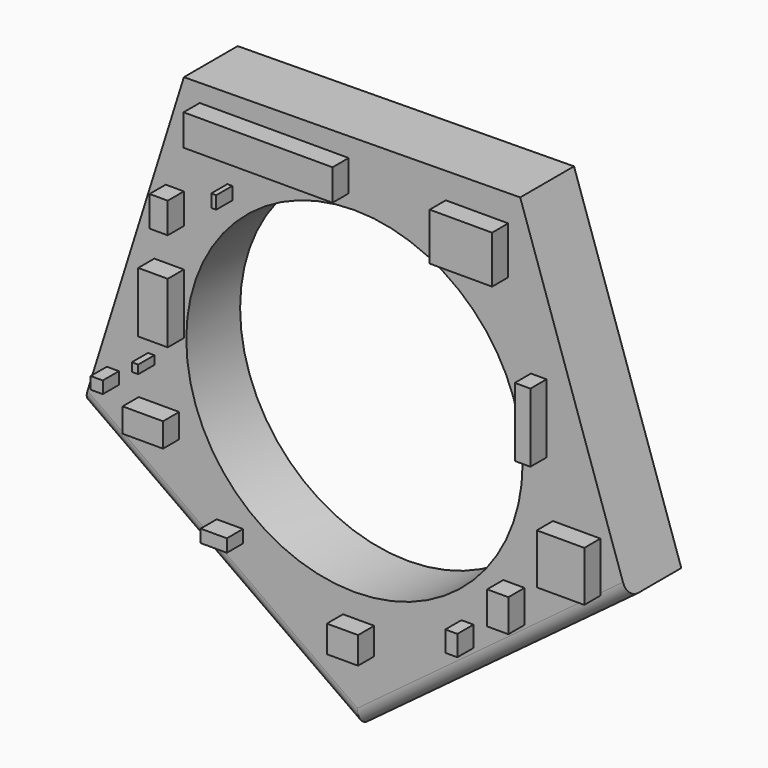
from build123d import *

# Parameters (mm, degrees)
F0_R         = 25
F1_DEPTH     = 10
F2_W         = 0.9488426149
F2_H         = 1.2651239522
F2_W_2       = 6.0093384236
F2_H_2       = 3.584517166
F2_W_3       = 3.9007980376
F2_H_3       = 1.8976870924
F2_W_4       = 4.6387878247
F2_H_4       = 4.0062256157
F2_W_5       = 1.7922576517
F2_H_5       = 3.0573830009
F2_W_6       = 7.0636067539
F2_H_6       = 7.4619053196
F2_W_7       = 3.1628105789
F2_H_7       = 4.8496406525
F2_W_8       = 2.3193918169
F2_H_8       = 10.2264162851
F2_W_9       = 9.2775728554
F2_H_9       = 7.0636067539
F2_W_10      = 22.1396633424
F2_H_10      = 4.6387854964
F2_W_11      = 2.7022243196
F2_H_11      = 4.5333597809
F2_W_12      = 0.7379893214
F2_H_12      = 1.8976833671
F2_W_13      = 4.3890562559
F2_H_13      = 8.9737139642
F2_W_14      = 1.7922595143
F2_H_14      = 1.7922581173
F3_DEPTH     = 3
F4_T1_DEPTH  = 60
F4_T6_DEPTH  = 60
F4_T12_DEPTH = 60
F4_T18_DEPTH = 60


# Not quite as in the source:
# - a fillet or chamfer that OpenCascade refuses, or shapes differently, is made with other operations: its cross-section is extruded or revolved along the edge and cut away or added


with BuildPart() as f1:
    # F0 (on Front) → F1 (new body)
    with BuildSketch(Plane.XZ):
        Polygon((-25.3573476618, 34.1470630352), (-40.3116381718, -13.5642479438), (0.4433851295, -42.5302292964), (40.5856652519, -12.7208793106), (24.6399354522, 34.6682935156), align=None)
        Circle(F0_R, mode=Mode.SUBTRACT)
    extrude(amount=F1_DEPTH)

    # F2 (on face) → F3 (join)
    with BuildSketch(Plane.XZ.offset(10)):
        with Locations((-30.2208252251, -4.310084274)):
            Rectangle(F2_W, F2_H)
        with Locations((-29.0611283854, -11.6899730638)):
            Rectangle(F2_W_2, F2_H_2)
        with Locations((-18.5184301808, -23.0760863051)):
            Rectangle(F2_W_3, F2_H_3)
        with Locations((0.6165653467, -30.455974862)):
            Rectangle(F2_W_4, F2_H_4)
        with Locations((16.7996054515, -25.0264853239)):
            Rectangle(F2_W_5, F2_H_5)
        with Locations((33.0353630707, -9.833295284)):
            Rectangle(F2_W_6, F2_H_6)
        with Locations((23.7050717697, -18.6481522396)):
            Rectangle(F2_W_7, F2_H_7)
        with Locations((27.3950155824, 7.0233154693)):
            Rectangle(F2_W_8, F2_H_8)
        with Locations((18.2228693739, 27.1598668769)):
            Rectangle(F2_W_9, F2_H_9)
        with Locations((-11.9292445015, 29.2156925425)):
            Rectangle(F2_W_10, F2_H_10)
        with Locations((-26.7084598216, 16.9334514067)):
            Rectangle(F2_W_11, F2_H_11)
        with Locations((-18.5184301808, 21.3086707518)):
            Rectangle(F2_W_12, F2_H_12)
        with Locations((-27.5518757897, 4.4868569821)):
            Rectangle(F2_W_13, F2_H_13)
        with Locations((-35.9138809144, -8.3690227475)):
            Rectangle(F2_W_14, F2_H_14)
    extrude(amount=F3_DEPTH)

    # F4: fillet of radius 2 on 2 edges, made by hand

    # F4_s2 → F4_t1 (cut)
    with BuildSketch(Plane(origin=(-24.4530139807, 0, 17.3795888115), x_dir=(0, 1, 0), z_dir=(0.815100466, 0, -0.5793196271))):
        with BuildLine():
            ThreePointArc((-8, -34.4095480118), (-9.4142135624, -33.8237615742), (-10, -32.4095480118))
            Line((-10, -32.4095480118), (-10, -34.4095480118))
            Line((-10, -34.4095480118), (-8, -34.4095480118))
        make_face()
    extrude(amount=F4_T1_DEPTH, mode=Mode.SUBTRACT)


with BuildPart() as f4_tool4:
    # F4_s5 → F4_t6 (new body)
    with BuildSketch(Plane(origin=(-24.0853680735, 0, -17.8856099914), x_dir=(0, 1, 0), z_dir=(0.8028456024, 0, 0.5961869997))):
        with BuildLine():
            ThreePointArc((-10, -32.4095480118), (-9.4142135624, -33.8237615742), (-8, -34.4095480118))
            Line((-8, -34.4095480118), (-10, -34.4095480118))
            Line((-10, -34.4095480118), (-10, -32.4095480118))
        make_face()
    extrude(amount=F4_T6_DEPTH)

    split(bisect_by=Plane.XY.offset(-13.5642479438), keep=Keep.BOTTOM)

    split(bisect_by=Plane.YZ.offset(36.5671664476), keep=Keep.BOTTOM)


with BuildPart() as f1_1:
    add(f1.part)

    # F4_t3: cut F4_tool4
    add(f4_tool4.part, mode=Mode.SUBTRACT)


with BuildPart() as f4_tool10:
    # F4_s11 → F4_t12 (new body)
    with BuildSketch(Plane(origin=(-24.0853680735, 0, -17.8856099914), x_dir=(0, 1, 0), z_dir=(0.8028456024, 0, 0.5961869997))):
        with BuildLine():
            ThreePointArc((-10, -32.4095480118), (-9.4142135624, -33.8237615742), (-8, -34.4095480118))
            Line((-8, -34.4095480118), (-10, -34.4095480118))
            Line((-10, -34.4095480118), (-10, -32.4095480118))
        make_face()
    extrude(amount=F4_T12_DEPTH)

    split(bisect_by=Plane.XY.offset(-13.5642479438), keep=Keep.BOTTOM)

    split(bisect_by=Plane.YZ.offset(36.5671664476), keep=Keep.TOP)


with BuildPart() as f1_2:
    add(f1_1.part)

    # F4_t9: cut F4_tool10
    add(f4_tool10.part, mode=Mode.SUBTRACT)


with BuildPart() as f4_tool16:
    # F4_s17 → F4_t18 (new body)
    with BuildSketch(Plane(origin=(-24.0853680735, 0, -17.8856099914), x_dir=(0, 1, 0), z_dir=(0.8028456024, 0, 0.5961869997))):
        with BuildLine():
            ThreePointArc((-10, -32.4095480118), (-9.4142135624, -33.8237615742), (-8, -34.4095480118))
            Line((-8, -34.4095480118), (-10, -34.4095480118))
            Line((-10, -34.4095480118), (-10, -32.4095480118))
        make_face()
    extrude(amount=F4_T18_DEPTH)

    split(bisect_by=Plane.XY.offset(-13.5642479438), keep=Keep.TOP)

    split(bisect_by=Plane.YZ.offset(36.5671664476), keep=Keep.TOP)


with BuildPart() as f1_3:
    add(f1_2.part)

    # F4_t15: cut F4_tool16
    add(f4_tool16.part, mode=Mode.SUBTRACT)


solid = f1_3.part
